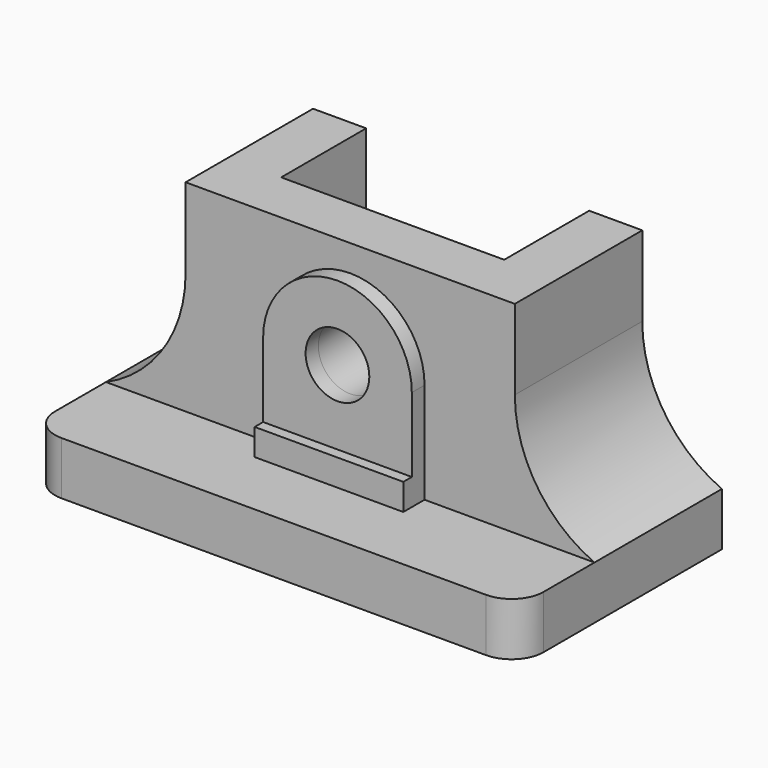
from build123d import *

# Parameters (mm, degrees)
F1_DEPTH    = 48
F2_DEPTH    = 10
F3_R        = 6
F4_T1_DEPTH = 30
F5_T1_DEPTH = 30
F7_DEPTH    = 5
F6_R        = 6
F8_DEPTH    = 3
F9_DEPTH    = 25


# Not quite as in the source:
# - a fillet or chamfer that OpenCascade refuses, or shapes differently, is made with other operations: its cross-section is extruded or revolved along the edge and cut away or added


with BuildPart() as f1:
    # F0 (on Top) → F1 (new body)
    with BuildSketch(Plane.XY):
        Polygon((21, 11.6292974651), (0, 11.6292974651), (-21, 11.6292974651), (-21, 31.6292974651), (-31, 31.6292974651), (-31, 1.6292974651), (0, 1.6292974651), (31, 1.6292974651), (31, 31.6292974651), (21, 31.6292974651), align=None)
    extrude(amount=F1_DEPTH)

    # F0 (on Top) → F2 (join)
    with BuildSketch(Plane.XY):
        Polygon((21, 11.6292974651), (0, 11.6292974651), (-21, 11.6292974651), (-21, 31.6292974651), (-31, 31.6292974651), (-31, 1.6292974651), (0, 1.6292974651), (31, 1.6292974651), (31, 31.6292974651), (21, 31.6292974651), align=None)
        Polygon((-31, 1.6292974651), (-31, 31.6292974651), (-46, 31.6292974651), (-46, -16.3707025349), (0, -16.3707025349), (46, -16.3707025349), (46, 31.6292974651), (31, 31.6292974651), (31, 1.6292974651), (0, 1.6292974651), align=None)
    extrude(amount=F2_DEPTH)

    # F3
    f3_edges = [f1.edges().sort_by_distance(p)[0] for p in [
        (-46, -16.370703, 5),
        (46, -16.370703, 5),
    ]]
    fillet(f3_edges, radius=F3_R)

    # F4: fillet of radius 25 on 1 edges, made by hand

    # F4_s2 → F4_t1 (join)
    with BuildSketch(Plane.XZ.offset(-31.6292974651)):
        with BuildLine():
            ThreePointArc((-46, 10), (-35.0834993366, 19.2198145372), (-31, 32.9128784748))
            Line((-31, 32.9128784748), (-31, 10))
            Line((-31, 10), (-46, 10))
        make_face()
    extrude(amount=F4_T1_DEPTH)

    # F5: fillet of radius 25 on 1 edges, made by hand

    # F5_s2 → F5_t1 (join)
    with BuildSketch(Plane.XZ.offset(-31.6292974651)):
        with BuildLine():
            ThreePointArc((46, 10), (35.0834993366, 19.2198145372), (31, 32.9128784748))
            Line((31, 32.9128784748), (31, 10))
            Line((31, 10), (46, 10))
        make_face()
    extrude(amount=F5_T1_DEPTH)

    # F6 (on face) → F7 (join)
    with BuildSketch(Plane.XZ.offset(-1.6292974651)):
        Polygon((14, 15), (0, 15), (-14, 15), (-14, 10), (14, 10), align=None)
    extrude(amount=F7_DEPTH)

    # F6 (on face) → F8 (join)
    with BuildSketch(Plane.XZ.offset(-1.6292974651)):
        with BuildLine():
            ThreePointArc((0, 15), (9.8994949366, 19.1005050634), (14, 29))
            ThreePointArc((14, 29), (0, 43), (-14, 29))
            ThreePointArc((-14, 29), (-9.8994949366, 19.1005050634), (0, 15))
        make_face()
        with Locations((0, 29)):
            Circle(F6_R, mode=Mode.SUBTRACT)
        with BuildLine():
            Line((14, 15), (14, 29))
            ThreePointArc((14, 29), (9.8994949366, 19.1005050634), (0, 15))
            Line((0, 15), (14, 15))
        make_face()
        with BuildLine():
            ThreePointArc((0, 15), (-9.8994949366, 19.1005050634), (-14, 29))
            Line((-14, 29), (-14, 15))
            Line((-14, 15), (0, 15))
        make_face()
        Polygon((14, 15), (0, 15), (-14, 15), (-14, 10), (14, 10), align=None)
    extrude(amount=F8_DEPTH)

    # F9 (cut): a face of the model
    f9_faces = [f1.faces().sort_by_distance(p)[0] for p in [
        (0, 1.6292974651, 29),
    ]]
    extrude(f9_faces, amount=-F9_DEPTH, mode=Mode.SUBTRACT)


solid = f1.part
